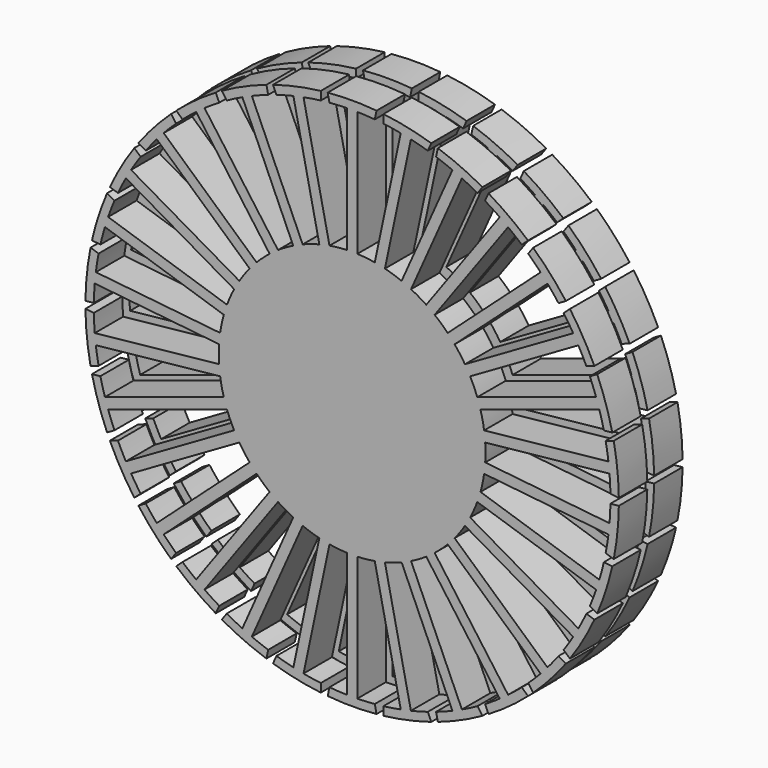
from build123d import *

# Parameters (mm, degrees)
F1_DEPTH = 25.4
F2_R     = 86.282686122
F3_DEPTH = 6.35
F5_DEPTH = 25.4


# Not quite as in the source:
# - a feature names something its author has since deleted; it is built from what else it names


with BuildPart() as f1:
    # F0 (on Front) → F1 (new body)
    with BuildSketch(Plane.XZ):
        with BuildLine():
            Line((16.1989831222, 183.765304664), (17.4450667429, 189.6995509914))
            ThreePointArc((17.4450667429, 189.6995509914), (0, 190.5), (-17.4450667429, 189.6995509914))
            Line((-17.4450667429, 189.6995509914), (-16.1989831222, 183.765304664))
            ThreePointArc((-16.1989831222, 183.765304664), (-9.9568666377, 184.2089983122), (-3.7032927424, 184.4407218466))
            Line((-3.7032927424, 184.4407218466), (-3.7032927424, 95.1779812922))
            ThreePointArc((-3.7032927424, 95.1779812922), (-9.9563361262, 94.7282105338), (-16.1662481083, 93.8680718993))
            ThreePointArc((-16.1662481083, 93.8680718993), (-19.8035885504, 93.1685589699), (-23.4109819298, 92.328156188))
            ThreePointArc((-23.4109819298, 92.328156188), (-29.4338687142, 90.5881331771), (-35.3292463424, 88.4556773355))
            ThreePointArc((-35.3292463424, 88.4556773355), (-38.741665253, 87.0152048405), (-42.0954988686, 85.4431476188))
            ThreePointArc((-42.0954988686, 85.4431476188), (-47.625, 82.4889197105), (-52.9481869828, 79.1773452146))
            ThreePointArc((-52.9481869828, 79.1773452146), (-55.9865452809, 77.0588687142), (-58.9402405103, 74.8238634968))
            ThreePointArc((-58.9402405103, 74.8238634968), (-63.7346902557, 70.7845446267), (-68.2530377785, 66.4385831728))
            ThreePointArc((-68.2530377785, 66.4385831728), (-70.7845446267, 63.7346902557), (-73.2090108149, 60.9344174954))
            ThreePointArc((-73.2090108149, 60.9344174954), (-77.0588687142, 55.9865452809), (-80.5749033088, 50.7961362387))
            ThreePointArc((-80.5749033088, 50.7961362387), (-82.4889197105, 47.625), (-84.2781960512, 44.3818450536))
            ThreePointArc((-84.2781960512, 44.3818450536), (-87.0152048405, 38.741665253), (-89.3752589233, 32.933654404))
            ThreePointArc((-89.3752589233, 32.933654404), (-90.5881331771, 29.4338687142), (-91.6640197083, 25.8895730152))
            ThreePointArc((-91.6640197083, 25.8895730152), (-93.1685589699, 19.8035885504), (-94.2694868527, 13.6318138386))
            ThreePointArc((-94.2694868527, 13.6318138386), (-94.7282105338, 9.9563361262), (-95.0436858515, 6.2658024042))
            ThreePointArc((-95.0436858515, 6.2658024042), (-95.25, 0), (-95.0436858515, -6.2658024042))
            ThreePointArc((-95.0436858515, -6.2658024042), (-94.7282105338, -9.9563361262), (-94.2694868527, -13.6318138386))
            ThreePointArc((-94.2694868527, -13.6318138386), (-93.1685589699, -19.8035885504), (-91.6640197083, -25.8895730152))
            ThreePointArc((-91.6640197083, -25.8895730152), (-90.5881331771, -29.4338687142), (-89.3752589233, -32.933654404))
            ThreePointArc((-89.3752589233, -32.933654404), (-87.0152048405, -38.741665253), (-84.2781960512, -44.3818450536))
            ThreePointArc((-84.2781960512, -44.3818450536), (-82.4889197105, -47.625), (-80.5749033088, -50.7961362387))
            ThreePointArc((-80.5749033088, -50.7961362387), (-77.0588687142, -55.9865452809), (-73.2090108149, -60.9344174954))
            ThreePointArc((-73.2090108149, -60.9344174954), (-70.7845446267, -63.7346902557), (-68.2530377785, -66.4385831728))
            ThreePointArc((-68.2530377785, -66.4385831728), (-63.7346902557, -70.7845446267), (-58.9402405103, -74.8238634968))
            ThreePointArc((-58.9402405103, -74.8238634968), (-55.9865452809, -77.0588687142), (-52.9481869828, -79.1773452146))
            ThreePointArc((-52.9481869828, -79.1773452146), (-47.625, -82.4889197105), (-42.0954988686, -85.4431476188))
            ThreePointArc((-42.0954988686, -85.4431476188), (-38.741665253, -87.0152048405), (-35.3292463424, -88.4556773355))
            ThreePointArc((-35.3292463424, -88.4556773355), (-29.4338687142, -90.5881331771), (-23.4109819298, -92.328156188))
            ThreePointArc((-23.4109819298, -92.328156188), (-19.8035885504, -93.1685589699), (-16.1662481083, -93.8680718993))
            ThreePointArc((-16.1662481083, -93.8680718993), (-9.9563361262, -94.7282105338), (-3.7032927424, -95.1779812922))
            ThreePointArc((-3.7032927424, -95.1779812922), (0, -95.25), (3.7032927424, -95.1779812922))
            ThreePointArc((3.7032927424, -95.1779812922), (9.9563361262, -94.7282105338), (16.1662481083, -93.8680718993))
            ThreePointArc((16.1662481083, -93.8680718993), (19.8035885504, -93.1685589699), (23.4109819298, -92.328156188))
            ThreePointArc((23.4109819298, -92.328156188), (29.4338687142, -90.5881331771), (35.3292463424, -88.4556773355))
            ThreePointArc((35.3292463424, -88.4556773355), (38.741665253, -87.0152048405), (42.0954988686, -85.4431476188))
            ThreePointArc((42.0954988686, -85.4431476188), (47.625, -82.4889197105), (52.9481869828, -79.1773452146))
            ThreePointArc((52.9481869828, -79.1773452146), (55.9865452809, -77.0588687142), (58.9402405103, -74.8238634968))
            ThreePointArc((58.9402405103, -74.8238634968), (63.7346902557, -70.7845446267), (68.2530377785, -66.4385831728))
            ThreePointArc((68.2530377785, -66.4385831728), (70.7845446267, -63.7346902557), (73.2090108149, -60.9344174954))
            ThreePointArc((73.2090108149, -60.9344174954), (77.0588687142, -55.9865452809), (80.5749033088, -50.7961362387))
            ThreePointArc((80.5749033088, -50.7961362387), (82.4889197105, -47.625), (84.2781960512, -44.3818450536))
            ThreePointArc((84.2781960512, -44.3818450536), (87.0152048405, -38.741665253), (89.3752589233, -32.933654404))
            ThreePointArc((89.3752589233, -32.933654404), (90.5881331771, -29.4338687142), (91.6640197083, -25.8895730152))
            ThreePointArc((91.6640197083, -25.8895730152), (93.1685589699, -19.8035885504), (94.2694868527, -13.6318138386))
            ThreePointArc((94.2694868527, -13.6318138386), (94.7282105338, -9.9563361262), (95.0436858515, -6.2658024042))
            ThreePointArc((95.0436858515, -6.2658024042), (95.25, 0), (95.0436858515, 6.2658024042))
            ThreePointArc((95.0436858515, 6.2658024042), (94.7282105338, 9.9563361262), (94.2694868527, 13.6318138386))
            ThreePointArc((94.2694868527, 13.6318138386), (93.1685589699, 19.8035885504), (91.6640197083, 25.8895730152))
            ThreePointArc((91.6640197083, 25.8895730152), (90.5881331771, 29.4338687142), (89.3752589233, 32.933654404))
            ThreePointArc((89.3752589233, 32.933654404), (87.0152048405, 38.741665253), (84.2781960512, 44.3818450536))
            ThreePointArc((84.2781960512, 44.3818450536), (82.4889197105, 47.625), (80.5749033088, 50.7961362387))
            ThreePointArc((80.5749033088, 50.7961362387), (77.0588687142, 55.9865452809), (73.2090108149, 60.9344174954))
            ThreePointArc((73.2090108149, 60.9344174954), (70.7845446267, 63.7346902557), (68.2530377785, 66.4385831728))
            ThreePointArc((68.2530377785, 66.4385831728), (63.7346902557, 70.7845446267), (58.9402405103, 74.8238634968))
            ThreePointArc((58.9402405103, 74.8238634968), (55.9865452809, 77.0588687142), (52.9481869828, 79.1773452146))
            ThreePointArc((52.9481869828, 79.1773452146), (47.625, 82.4889197105), (42.0954988686, 85.4431476188))
            ThreePointArc((42.0954988686, 85.4431476188), (38.741665253, 87.0152048405), (35.3292463424, 88.4556773355))
            ThreePointArc((35.3292463424, 88.4556773355), (29.4338687142, 90.5881331771), (23.4109819298, 92.328156188))
            ThreePointArc((23.4109819298, 92.328156188), (19.8035885504, 93.1685589699), (16.1662481083, 93.8680718993))
            ThreePointArc((16.1662481083, 93.8680718993), (9.9563361262, 94.7282105338), (3.7032927424, 95.1779812922))
            Line((3.7032927424, 95.1779812922), (3.7032927424, 184.4407218466))
            ThreePointArc((3.7032927424, 184.4407218466), (9.9568666377, 184.2089983122), (16.1989831222, 183.765304664))
        make_face()
        with BuildLine():
            ThreePointArc((-23.4109819298, 92.328156188), (-19.8035885504, 93.1685589699), (-16.1662481083, 93.8680718993))
            Line((-16.1662481083, 93.8680718993), (-34.725015424, 181.1802074075))
            ThreePointArc((-34.725015424, 181.1802074075), (-28.5599190905, 182.2537387106), (-22.361958731, 183.1175498257))
            Line((-22.361958731, 183.1175498257), (-22.3769042148, 189.1811939855))
            ThreePointArc((-22.3769042148, 189.1811939855), (-39.6071771008, 186.3371179398), (-56.5046045732, 181.9271273396))
            Line((-56.5046045732, 181.9271273396), (-54.0519516817, 176.3816338847))
            ThreePointArc((-54.0519516817, 176.3816338847), (-48.0384895154, 178.1134407548), (-41.9697492455, 179.6402916962))
            Line((-41.9697492455, 179.6402916962), (-23.4109819298, 92.328156188))
        make_face()
        with BuildLine():
            Line((34.725015424, 181.1802074075), (16.1662481083, 93.8680718993))
            ThreePointArc((16.1662481083, 93.8680718993), (19.8035885504, 93.1685589699), (23.4109819298, 92.328156188))
            Line((23.4109819298, 92.328156188), (41.9697492455, 179.6402916962))
            ThreePointArc((41.9697492455, 179.6402916962), (48.0384895154, 178.1134407548), (54.0519516817, 176.3816338847))
            Line((54.0519516817, 176.3816338847), (56.5046045732, 181.9271273396))
            ThreePointArc((56.5046045732, 181.9271273396), (39.6071771008, 186.3371179398), (22.3769042148, 189.1811939855))
            Line((22.3769042148, 189.1811939855), (22.361958731, 183.1175498257))
            ThreePointArc((22.361958731, 183.1175498257), (28.5599190905, 182.2537387106), (34.725015424, 181.1802074075))
        make_face()
        with BuildLine():
            Line((71.6356737873, 170.0012485057), (35.3292463424, 88.4556773355))
            ThreePointArc((35.3292463424, 88.4556773355), (38.741665253, 87.0152048405), (42.0954988686, 85.4431476188))
            Line((42.0954988686, 85.4431476188), (78.4019263135, 166.9887187889))
            ThreePointArc((78.4019263135, 166.9887187889), (84.0205998871, 164.2334711533), (89.5425905826, 161.2892393317))
            Line((89.5425905826, 161.2892393317), (93.0946200445, 166.2036152398))
            ThreePointArc((93.0946200445, 166.2036152398), (77.4833305059, 174.0304096809), (61.2208970819, 180.3947110103))
            Line((61.2208970819, 180.3947110103), (59.9455756831, 174.4666793645))
            ThreePointArc((59.9455756831, 174.4666793645), (65.8284993087, 172.3331161768), (71.6356737873, 170.0012485057))
        make_face()
        with BuildLine():
            Line((105.4155094599, 151.3924192876), (52.9481869828, 79.1773452146))
            ThreePointArc((52.9481869828, 79.1773452146), (55.9865452809, 77.0588687142), (58.9402405103, 74.8238634968))
            Line((58.9402405103, 74.8238634968), (111.4075629873, 147.0389375698))
            ThreePointArc((111.4075629873, 147.0389375698), (116.3306068681, 143.1757107827), (121.119788602, 139.1477310683))
            Line((121.119788602, 139.1477310683), (125.6159539023, 143.2162076206))
            ThreePointArc((125.6159539023, 143.2162076206), (111.9730905617, 154.1177374284), (97.3892429762, 163.7241135341))
            Line((97.3892429762, 163.7241135341), (94.909283327, 158.190777831))
            ThreePointArc((94.909283327, 158.190777831), (100.2200582269, 154.88070952), (105.4155094599, 151.3924192876))
        make_face()
        with BuildLine():
            Line((134.5881815294, 126.1670148852), (68.2530377785, 66.4385831728))
            ThreePointArc((68.2530377785, 66.4385831728), (70.7845446267, 63.7346902557), (73.2090108149, 60.9344174954))
            Line((73.2090108149, 60.9344174954), (139.5441545659, 120.6628492078))
            ThreePointArc((139.5441545659, 120.6628492078), (143.5564081128, 115.8604848177), (147.4034706623, 110.9247992522))
            Line((147.4034706623, 110.9247992522), (152.6472678023, 113.9695645008))
            ThreePointArc((152.6472678023, 113.9695645008), (141.5690892534, 127.4693805114), (129.301211627, 139.897986661))
            Line((129.301211627, 139.897986661), (125.7249998643, 135.0011802228))
            ThreePointArc((125.7249998643, 135.0011802228), (130.2315196914, 130.6592726572), (134.5881815294, 126.1670148852))
        make_face()
        with BuildLine():
            Line((157.8787042403, 95.4275065158), (80.5749033088, 50.7961362387))
            ThreePointArc((80.5749033088, 50.7961362387), (82.4889197105, 47.625), (84.2781960512, 44.3818450536))
            Line((84.2781960512, 44.3818450536), (161.5819969827, 89.0132153308))
            ThreePointArc((161.5819969827, 89.0132153308), (164.5081054629, 83.4815997058), (167.2449137343, 77.8539214327))
            Line((167.2449137343, 77.8539214327), (173.0071636165, 79.7419045256))
            ThreePointArc((173.0071636165, 79.7419045256), (164.9778394209, 95.25), (155.5620968736, 109.9576464658))
            Line((155.5620968736, 109.9576464658), (151.0459306121, 105.9113832313))
            ThreePointArc((151.0459306121, 105.9113832313), (154.5512388252, 100.7273986064), (157.8787042403, 95.4275065158))
        make_face()
        with BuildLine():
            Line((174.2691699899, 60.5173581998), (89.3752589233, 32.933654404))
            ThreePointArc((89.3752589233, 32.933654404), (90.5881331771, 29.4338687142), (91.6640197083, 25.8895730152))
            Line((91.6640197083, 25.8895730152), (176.5579307749, 53.473276811))
            ThreePointArc((176.5579307749, 53.473276811), (178.2700092068, 47.4541680976), (179.776951546, 41.3804536619))
            Line((179.776951546, 41.3804536619), (185.8058162002, 42.0291406786))
            ThreePointArc((185.8058162002, 42.0291406786), (181.1762663542, 58.8677374284), (175.0241720171, 75.2116294847))
            Line((175.0241720171, 75.2116294847), (169.7654293933, 72.1927505734))
            ThreePointArc((169.7654293933, 72.1927505734), (172.1163272033, 66.3932538929), (174.2691699899, 60.5173581998))
        make_face()
        with BuildLine():
            Line((183.0432367746, 22.9623109358), (94.2694868527, 13.6318138386))
            ThreePointArc((94.2694868527, 13.6318138386), (94.7282105338, 9.9563361262), (95.0436858515, 6.2658024042))
            Line((95.0436858515, 6.2658024042), (183.8174357734, 15.5962995014))
            ThreePointArc((183.8174357734, 15.5962995014), (184.240658114, 9.3527616332), (184.4518739096, 3.0984615007))
            Line((184.4518739096, 3.0984615007), (190.4838630207, 2.4795017057))
            ThreePointArc((190.4838630207, 2.4795017057), (189.4564210677, 19.9126722525), (186.8368509842, 37.1785033897))
            Line((186.8368509842, 37.1785033897), (181.0653642851, 35.3189482962))
            ThreePointArc((181.0653642851, 35.3189482962), (182.1591061768, 29.1574053941), (183.0432367746, 22.9623109358))
        make_face()
        with BuildLine():
            Line((183.8174357734, -15.5962995014), (95.0436858515, -6.2658024042))
            ThreePointArc((95.0436858515, -6.2658024042), (94.7282105338, -9.9563361262), (94.2694868527, -13.6318138386))
            Line((94.2694868527, -13.6318138386), (183.0432367746, -22.9623109358))
            ThreePointArc((183.0432367746, -22.9623109358), (182.1591061768, -29.1574053941), (181.0653642851, -35.3189482962))
            Line((181.0653642851, -35.3189482962), (186.8368509842, -37.1785033897))
            ThreePointArc((186.8368509842, -37.1785033897), (189.4564210677, -19.9126722525), (190.4838630207, -2.4795017057))
            Line((190.4838630207, -2.4795017057), (184.4518739096, -3.0984615007))
            ThreePointArc((184.4518739096, -3.0984615007), (184.240658114, -9.3527616332), (183.8174357734, -15.5962995014))
        make_face()
        with BuildLine():
            Line((176.5579307749, -53.473276811), (91.6640197083, -25.8895730152))
            ThreePointArc((91.6640197083, -25.8895730152), (90.5881331771, -29.4338687142), (89.3752589233, -32.933654404))
            Line((89.3752589233, -32.933654404), (174.2691699899, -60.5173581998))
            ThreePointArc((174.2691699899, -60.5173581998), (172.1163272033, -66.3932538929), (169.7654293933, -72.1927505734))
            Line((169.7654293933, -72.1927505734), (175.0241720171, -75.2116294847))
            ThreePointArc((175.0241720171, -75.2116294847), (181.1762663542, -58.8677374284), (185.8058162002, -42.0291406786))
            Line((185.8058162002, -42.0291406786), (179.776951546, -41.3804536619))
            ThreePointArc((179.776951546, -41.3804536619), (178.2700092068, -47.4541680976), (176.5579307749, -53.473276811))
        make_face()
        with BuildLine():
            Line((161.5819969827, -89.0132153308), (84.2781960512, -44.3818450536))
            ThreePointArc((84.2781960512, -44.3818450536), (82.4889197105, -47.625), (80.5749033088, -50.7961362387))
            Line((80.5749033088, -50.7961362387), (157.8787042403, -95.4275065158))
            ThreePointArc((157.8787042403, -95.4275065158), (154.5512388252, -100.7273986064), (151.0459306121, -105.9113832313))
            Line((151.0459306121, -105.9113832313), (155.5620968736, -109.9576464658))
            ThreePointArc((155.5620968736, -109.9576464658), (164.9778394209, -95.25), (173.0071636165, -79.7419045256))
            Line((173.0071636165, -79.7419045256), (167.2449137343, -77.8539214327))
            ThreePointArc((167.2449137343, -77.8539214327), (164.5081054629, -83.4815997058), (161.5819969827, -89.0132153308))
        make_face()
        with BuildLine():
            Line((139.5441545659, -120.6628492078), (73.2090108149, -60.9344174954))
            ThreePointArc((73.2090108149, -60.9344174954), (70.7845446267, -63.7346902557), (68.2530377785, -66.4385831728))
            Line((68.2530377785, -66.4385831728), (134.5881815294, -126.1670148852))
            ThreePointArc((134.5881815294, -126.1670148852), (130.2315196914, -130.6592726572), (125.7249998643, -135.0011802228))
            Line((125.7249998643, -135.0011802228), (129.301211627, -139.897986661))
            ThreePointArc((129.301211627, -139.897986661), (141.5690892534, -127.4693805114), (152.6472678023, -113.9695645008))
            Line((152.6472678023, -113.9695645008), (147.4034706623, -110.9247992522))
            ThreePointArc((147.4034706623, -110.9247992522), (143.5564081128, -115.8604848177), (139.5441545659, -120.6628492078))
        make_face()
        with BuildLine():
            Line((111.4075629873, -147.0389375698), (58.9402405103, -74.8238634968))
            ThreePointArc((58.9402405103, -74.8238634968), (55.9865452809, -77.0588687142), (52.9481869828, -79.1773452146))
            Line((52.9481869828, -79.1773452146), (105.4155094599, -151.3924192876))
            ThreePointArc((105.4155094599, -151.3924192876), (100.2200582269, -154.88070952), (94.909283327, -158.190777831))
            Line((94.909283327, -158.190777831), (97.3892429762, -163.7241135341))
            ThreePointArc((97.3892429762, -163.7241135341), (111.9730905617, -154.1177374284), (125.6159539023, -143.2162076206))
            Line((125.6159539023, -143.2162076206), (121.119788602, -139.1477310683))
            ThreePointArc((121.119788602, -139.1477310683), (116.3306068681, -143.1757107827), (111.4075629873, -147.0389375698))
        make_face()
        with BuildLine():
            Line((78.4019263135, -166.9887187889), (42.0954988686, -85.4431476188))
            ThreePointArc((42.0954988686, -85.4431476188), (38.741665253, -87.0152048405), (35.3292463424, -88.4556773355))
            Line((35.3292463424, -88.4556773355), (71.6356737873, -170.0012485057))
            ThreePointArc((71.6356737873, -170.0012485057), (65.8284993087, -172.3331161768), (59.9455756831, -174.4666793645))
            Line((59.9455756831, -174.4666793645), (61.2208970819, -180.3947110103))
            ThreePointArc((61.2208970819, -180.3947110103), (77.4833305059, -174.0304096809), (93.0946200445, -166.2036152398))
            Line((93.0946200445, -166.2036152398), (89.5425905826, -161.2892393317))
            ThreePointArc((89.5425905826, -161.2892393317), (84.0205998871, -164.2334711533), (78.4019263135, -166.9887187889))
        make_face()
        with BuildLine():
            Line((41.9697492455, -179.6402916962), (23.4109819298, -92.328156188))
            ThreePointArc((23.4109819298, -92.328156188), (19.8035885504, -93.1685589699), (16.1662481083, -93.8680718993))
            Line((16.1662481083, -93.8680718993), (34.725015424, -181.1802074075))
            ThreePointArc((34.725015424, -181.1802074075), (28.5599190905, -182.2537387106), (22.361958731, -183.1175498257))
            Line((22.361958731, -183.1175498257), (22.3769042148, -189.1811939855))
            ThreePointArc((22.3769042148, -189.1811939855), (39.6071771008, -186.3371179398), (56.5046045732, -181.9271273396))
            Line((56.5046045732, -181.9271273396), (54.0519516817, -176.3816338847))
            ThreePointArc((54.0519516817, -176.3816338847), (48.0384895154, -178.1134407548), (41.9697492455, -179.6402916962))
        make_face()
        with BuildLine():
            Line((3.7032927424, -184.4407218466), (3.7032927424, -95.1779812922))
            ThreePointArc((3.7032927424, -95.1779812922), (0, -95.25), (-3.7032927424, -95.1779812922))
            Line((-3.7032927424, -95.1779812922), (-3.7032927424, -184.4407218466))
            ThreePointArc((-3.7032927424, -184.4407218466), (-9.9568666377, -184.2089983122), (-16.1989831222, -183.765304664))
            Line((-16.1989831222, -183.765304664), (-17.4450667429, -189.6995509914))
            ThreePointArc((-17.4450667429, -189.6995509914), (0, -190.5), (17.4450667429, -189.6995509914))
            Line((17.4450667429, -189.6995509914), (16.1989831222, -183.765304664))
            ThreePointArc((16.1989831222, -183.765304664), (9.9568666377, -184.2089983122), (3.7032927424, -184.4407218466))
        make_face()
        with BuildLine():
            ThreePointArc((-16.1662481083, -93.8680718993), (-19.8035885504, -93.1685589699), (-23.4109819298, -92.328156188))
            Line((-23.4109819298, -92.328156188), (-41.9697492455, -179.6402916962))
            ThreePointArc((-41.9697492455, -179.6402916962), (-48.0384895154, -178.1134407548), (-54.0519516817, -176.3816338847))
            Line((-54.0519516817, -176.3816338847), (-56.5046045732, -181.9271273396))
            ThreePointArc((-56.5046045732, -181.9271273396), (-39.6071771008, -186.3371179398), (-22.3769042148, -189.1811939855))
            Line((-22.3769042148, -189.1811939855), (-22.361958731, -183.1175498257))
            ThreePointArc((-22.361958731, -183.1175498257), (-28.5599190905, -182.2537387106), (-34.725015424, -181.1802074075))
            Line((-34.725015424, -181.1802074075), (-16.1662481083, -93.8680718993))
        make_face()
        with BuildLine():
            ThreePointArc((-35.3292463424, -88.4556773355), (-38.741665253, -87.0152048405), (-42.0954988686, -85.4431476188))
            Line((-42.0954988686, -85.4431476188), (-78.4019263135, -166.9887187889))
            ThreePointArc((-78.4019263135, -166.9887187889), (-84.0205998871, -164.2334711533), (-89.5425905826, -161.2892393317))
            Line((-89.5425905826, -161.2892393317), (-93.0946200445, -166.2036152398))
            ThreePointArc((-93.0946200445, -166.2036152398), (-77.4833305059, -174.0304096809), (-61.2208970819, -180.3947110103))
            Line((-61.2208970819, -180.3947110103), (-59.9455756831, -174.4666793645))
            ThreePointArc((-59.9455756831, -174.4666793645), (-65.8284993087, -172.3331161768), (-71.6356737873, -170.0012485057))
            Line((-71.6356737873, -170.0012485057), (-35.3292463424, -88.4556773355))
        make_face()
        with BuildLine():
            ThreePointArc((-52.9481869828, -79.1773452146), (-55.9865452809, -77.0588687142), (-58.9402405103, -74.8238634968))
            Line((-58.9402405103, -74.8238634968), (-111.4075629873, -147.0389375698))
            ThreePointArc((-111.4075629873, -147.0389375698), (-116.3306068681, -143.1757107827), (-121.119788602, -139.1477310683))
            Line((-121.119788602, -139.1477310683), (-125.6159539023, -143.2162076206))
            ThreePointArc((-125.6159539023, -143.2162076206), (-111.9730905617, -154.1177374284), (-97.3892429762, -163.7241135341))
            Line((-97.3892429762, -163.7241135341), (-94.909283327, -158.190777831))
            ThreePointArc((-94.909283327, -158.190777831), (-100.2200582269, -154.88070952), (-105.4155094599, -151.3924192876))
            Line((-105.4155094599, -151.3924192876), (-52.9481869828, -79.1773452146))
        make_face()
        with BuildLine():
            ThreePointArc((-68.2530377785, -66.4385831728), (-70.7845446267, -63.7346902557), (-73.2090108149, -60.9344174954))
            Line((-73.2090108149, -60.9344174954), (-139.5441545659, -120.6628492078))
            ThreePointArc((-139.5441545659, -120.6628492078), (-143.5564081128, -115.8604848177), (-147.4034706623, -110.9247992522))
            Line((-147.4034706623, -110.9247992522), (-152.6472678023, -113.9695645008))
            ThreePointArc((-152.6472678023, -113.9695645008), (-141.5690892534, -127.4693805114), (-129.301211627, -139.897986661))
            Line((-129.301211627, -139.897986661), (-125.7249998643, -135.0011802228))
            ThreePointArc((-125.7249998643, -135.0011802228), (-130.2315196914, -130.6592726572), (-134.5881815294, -126.1670148852))
            Line((-134.5881815294, -126.1670148852), (-68.2530377785, -66.4385831728))
        make_face()
        with BuildLine():
            ThreePointArc((-80.5749033088, -50.7961362387), (-82.4889197105, -47.625), (-84.2781960512, -44.3818450536))
            Line((-84.2781960512, -44.3818450536), (-161.5819969827, -89.0132153308))
            ThreePointArc((-161.5819969827, -89.0132153308), (-164.5081054629, -83.4815997058), (-167.2449137343, -77.8539214327))
            Line((-167.2449137343, -77.8539214327), (-173.0071636165, -79.7419045256))
            ThreePointArc((-173.0071636165, -79.7419045256), (-164.9778394209, -95.25), (-155.5620968736, -109.9576464658))
            Line((-155.5620968736, -109.9576464658), (-151.0459306121, -105.9113832313))
            ThreePointArc((-151.0459306121, -105.9113832313), (-154.5512388252, -100.7273986064), (-157.8787042403, -95.4275065158))
            Line((-157.8787042403, -95.4275065158), (-80.5749033088, -50.7961362387))
        make_face()
        with BuildLine():
            ThreePointArc((-89.3752589233, -32.933654404), (-90.5881331771, -29.4338687142), (-91.6640197083, -25.8895730152))
            Line((-91.6640197083, -25.8895730152), (-176.5579307749, -53.473276811))
            ThreePointArc((-176.5579307749, -53.473276811), (-178.2700092068, -47.4541680976), (-179.776951546, -41.3804536619))
            Line((-179.776951546, -41.3804536619), (-185.8058162002, -42.0291406786))
            ThreePointArc((-185.8058162002, -42.0291406786), (-181.1762663542, -58.8677374284), (-175.0241720171, -75.2116294847))
            Line((-175.0241720171, -75.2116294847), (-169.7654293933, -72.1927505734))
            ThreePointArc((-169.7654293933, -72.1927505734), (-172.1163272033, -66.3932538929), (-174.2691699899, -60.5173581998))
            Line((-174.2691699899, -60.5173581998), (-89.3752589233, -32.933654404))
        make_face()
        with BuildLine():
            ThreePointArc((-94.2694868527, -13.6318138386), (-94.7282105338, -9.9563361262), (-95.0436858515, -6.2658024042))
            Line((-95.0436858515, -6.2658024042), (-183.8174357734, -15.5962995014))
            ThreePointArc((-183.8174357734, -15.5962995014), (-184.240658114, -9.3527616332), (-184.4518739096, -3.0984615007))
            Line((-184.4518739096, -3.0984615007), (-190.4838630207, -2.4795017057))
            ThreePointArc((-190.4838630207, -2.4795017057), (-189.4564210677, -19.9126722525), (-186.8368509842, -37.1785033897))
            Line((-186.8368509842, -37.1785033897), (-181.0653642851, -35.3189482962))
            ThreePointArc((-181.0653642851, -35.3189482962), (-182.1591061768, -29.1574053941), (-183.0432367746, -22.9623109358))
            Line((-183.0432367746, -22.9623109358), (-94.2694868527, -13.6318138386))
        make_face()
        with BuildLine():
            ThreePointArc((-95.0436858515, 6.2658024042), (-94.7282105338, 9.9563361262), (-94.2694868527, 13.6318138386))
            Line((-94.2694868527, 13.6318138386), (-183.0432367746, 22.9623109358))
            ThreePointArc((-183.0432367746, 22.9623109358), (-182.1591061768, 29.1574053941), (-181.0653642851, 35.3189482962))
            Line((-181.0653642851, 35.3189482962), (-186.8368509842, 37.1785033897))
            ThreePointArc((-186.8368509842, 37.1785033897), (-189.4564210677, 19.9126722525), (-190.4838630207, 2.4795017057))
            Line((-190.4838630207, 2.4795017057), (-184.4518739096, 3.0984615007))
            ThreePointArc((-184.4518739096, 3.0984615007), (-184.240658114, 9.3527616332), (-183.8174357734, 15.5962995014))
            Line((-183.8174357734, 15.5962995014), (-95.0436858515, 6.2658024042))
        make_face()
        with BuildLine():
            ThreePointArc((-91.6640197083, 25.8895730152), (-90.5881331771, 29.4338687142), (-89.3752589233, 32.933654404))
            Line((-89.3752589233, 32.933654404), (-174.2691699899, 60.5173581998))
            ThreePointArc((-174.2691699899, 60.5173581998), (-172.1163272033, 66.3932538929), (-169.7654293933, 72.1927505734))
            Line((-169.7654293933, 72.1927505734), (-175.0241720171, 75.2116294847))
            ThreePointArc((-175.0241720171, 75.2116294847), (-181.1762663542, 58.8677374284), (-185.8058162002, 42.0291406786))
            Line((-185.8058162002, 42.0291406786), (-179.776951546, 41.3804536619))
            ThreePointArc((-179.776951546, 41.3804536619), (-178.2700092068, 47.4541680976), (-176.5579307749, 53.473276811))
            Line((-176.5579307749, 53.473276811), (-91.6640197083, 25.8895730152))
        make_face()
        with BuildLine():
            ThreePointArc((-84.2781960512, 44.3818450536), (-82.4889197105, 47.625), (-80.5749033088, 50.7961362387))
            Line((-80.5749033088, 50.7961362387), (-157.8787042403, 95.4275065158))
            ThreePointArc((-157.8787042403, 95.4275065158), (-154.5512388252, 100.7273986064), (-151.0459306121, 105.9113832313))
            Line((-151.0459306121, 105.9113832313), (-155.5620968736, 109.9576464658))
            ThreePointArc((-155.5620968736, 109.9576464658), (-164.9778394209, 95.25), (-173.0071636165, 79.7419045256))
            Line((-173.0071636165, 79.7419045256), (-167.2449137343, 77.8539214327))
            ThreePointArc((-167.2449137343, 77.8539214327), (-164.5081054629, 83.4815997058), (-161.5819969827, 89.0132153308))
            Line((-161.5819969827, 89.0132153308), (-84.2781960512, 44.3818450536))
        make_face()
        with BuildLine():
            ThreePointArc((-73.2090108149, 60.9344174954), (-70.7845446267, 63.7346902557), (-68.2530377785, 66.4385831728))
            Line((-68.2530377785, 66.4385831728), (-134.5881815294, 126.1670148852))
            ThreePointArc((-134.5881815294, 126.1670148852), (-130.2315196914, 130.6592726572), (-125.7249998643, 135.0011802228))
            Line((-125.7249998643, 135.0011802228), (-129.301211627, 139.897986661))
            ThreePointArc((-129.301211627, 139.897986661), (-141.5690892534, 127.4693805114), (-152.6472678023, 113.9695645008))
            Line((-152.6472678023, 113.9695645008), (-147.4034706623, 110.9247992522))
            ThreePointArc((-147.4034706623, 110.9247992522), (-143.5564081128, 115.8604848177), (-139.5441545659, 120.6628492078))
            Line((-139.5441545659, 120.6628492078), (-73.2090108149, 60.9344174954))
        make_face()
        with BuildLine():
            ThreePointArc((-58.9402405103, 74.8238634968), (-55.9865452809, 77.0588687142), (-52.9481869828, 79.1773452146))
            Line((-52.9481869828, 79.1773452146), (-105.4155094599, 151.3924192876))
            ThreePointArc((-105.4155094599, 151.3924192876), (-100.2200582269, 154.88070952), (-94.909283327, 158.190777831))
            Line((-94.909283327, 158.190777831), (-97.3892429762, 163.7241135341))
            ThreePointArc((-97.3892429762, 163.7241135341), (-111.9730905617, 154.1177374284), (-125.6159539023, 143.2162076206))
            Line((-125.6159539023, 143.2162076206), (-121.119788602, 139.1477310683))
            ThreePointArc((-121.119788602, 139.1477310683), (-116.3306068681, 143.1757107827), (-111.4075629873, 147.0389375698))
            Line((-111.4075629873, 147.0389375698), (-58.9402405103, 74.8238634968))
        make_face()
        with BuildLine():
            ThreePointArc((-42.0954988686, 85.4431476188), (-38.741665253, 87.0152048405), (-35.3292463424, 88.4556773355))
            Line((-35.3292463424, 88.4556773355), (-71.6356737873, 170.0012485057))
            ThreePointArc((-71.6356737873, 170.0012485057), (-65.8284993087, 172.3331161768), (-59.9455756831, 174.4666793645))
            Line((-59.9455756831, 174.4666793645), (-61.2208970819, 180.3947110103))
            ThreePointArc((-61.2208970819, 180.3947110103), (-77.4833305059, 174.0304096809), (-93.0946200445, 166.2036152398))
            Line((-93.0946200445, 166.2036152398), (-89.5425905826, 161.2892393317))
            ThreePointArc((-89.5425905826, 161.2892393317), (-84.0205998871, 164.2334711533), (-78.4019263135, 166.9887187889))
            Line((-78.4019263135, 166.9887187889), (-42.0954988686, 85.4431476188))
        make_face()
    extrude(amount=F1_DEPTH)

    # F2 (on face) → F3 (join)
    with BuildSketch(Plane.XZ.offset(25.4)):
        Circle(F2_R)
    extrude(amount=F3_DEPTH)

    # F4 (on face) → F5 (join)
    with BuildSketch(Plane.XZ.offset(31.75)):
        with BuildLine():
            Line((16.3894969565, 182.7363048395), (17.6355805772, 188.6705511669))
            ThreePointArc((17.6355805772, 188.6705511669), (0.1905138342, 189.4710001755), (-17.2545529087, 188.6705511669))
            Line((-17.2545529087, 188.6705511669), (-16.008469288, 182.7363048395))
            ThreePointArc((-16.008469288, 182.7363048395), (-9.7663528034, 183.1799984878), (-3.5127789081, 183.4117220222))
            Line((-3.5127789081, 183.4117220222), (-3.5127789081, 94.1489814678))
            ThreePointArc((-3.5127789081, 94.1489814678), (-9.765822292, 93.6992107094), (-15.9757342741, 92.8390720749))
            ThreePointArc((-15.9757342741, 92.8390720749), (-19.6130747162, 92.1395591454), (-23.2204680956, 91.2991563636))
            ThreePointArc((-23.2204680956, 91.2991563636), (-29.24335488, 89.5591333527), (-35.1387325082, 87.426677511))
            ThreePointArc((-35.1387325082, 87.426677511), (-38.5511514187, 85.986205016), (-41.9049850344, 84.4141477943))
            ThreePointArc((-41.9049850344, 84.4141477943), (-47.4344861658, 81.459919886), (-52.7576731486, 78.1483453901))
            ThreePointArc((-52.7576731486, 78.1483453901), (-55.7960314466, 76.0298688898), (-58.749726676, 73.7948636724))
            ThreePointArc((-58.749726676, 73.7948636724), (-63.5441764214, 69.7555448023), (-68.0625239442, 65.4095833483))
            ThreePointArc((-68.0625239442, 65.4095833483), (-70.5940307925, 62.7056904312), (-73.0184969807, 59.9054176709))
            ThreePointArc((-73.0184969807, 59.9054176709), (-76.86835488, 54.9575454564), (-80.3843894746, 49.7671364142))
            ThreePointArc((-80.3843894746, 49.7671364142), (-82.2984058762, 46.5960001755), (-84.0876822169, 43.3528452291))
            ThreePointArc((-84.0876822169, 43.3528452291), (-86.8246910062, 37.7126654285), (-89.184745089, 31.9046545795))
            ThreePointArc((-89.184745089, 31.9046545795), (-90.3976193429, 28.4048688898), (-91.4735058741, 24.8605731908))
            ThreePointArc((-91.4735058741, 24.8605731908), (-92.9780451357, 18.7745887259), (-94.0789730184, 12.6028140142))
            ThreePointArc((-94.0789730184, 12.6028140142), (-94.5376966996, 8.9273363018), (-94.8531720172, 5.2368025797))
            ThreePointArc((-94.8531720172, 5.2368025797), (-95.0594861658, -1.0289998245), (-94.8531720172, -7.2948022286))
            ThreePointArc((-94.8531720172, -7.2948022286), (-94.5376966996, -10.9853359507), (-94.0789730184, -14.6608136631))
            ThreePointArc((-94.0789730184, -14.6608136631), (-92.9780451357, -20.8325883748), (-91.4735058741, -26.9185728397))
            ThreePointArc((-91.4735058741, -26.9185728397), (-90.3976193429, -30.4628685387), (-89.184745089, -33.9626542284))
            ThreePointArc((-89.184745089, -33.9626542284), (-86.8246910062, -39.7706650774), (-84.0876822169, -45.410844878))
            ThreePointArc((-84.0876822169, -45.410844878), (-82.2984058762, -48.6539998245), (-80.3843894746, -51.8251360631))
            ThreePointArc((-80.3843894746, -51.8251360631), (-76.86835488, -57.0155451053), (-73.0184969807, -61.9634173198))
            ThreePointArc((-73.0184969807, -61.9634173198), (-70.5940307925, -64.7636900801), (-68.0625239442, -67.4675829972))
            ThreePointArc((-68.0625239442, -67.4675829972), (-63.5441764214, -71.8135444512), (-58.749726676, -75.8528633213))
            ThreePointArc((-58.749726676, -75.8528633213), (-55.7960314466, -78.0878685387), (-52.7576731486, -80.2063450391))
            ThreePointArc((-52.7576731486, -80.2063450391), (-47.4344861658, -83.5179195349), (-41.9049850344, -86.4721474432))
            ThreePointArc((-41.9049850344, -86.4721474432), (-38.5511514187, -88.0442046649), (-35.1387325082, -89.4846771599))
            ThreePointArc((-35.1387325082, -89.4846771599), (-29.24335488, -91.6171330016), (-23.2204680956, -93.3571560125))
            ThreePointArc((-23.2204680956, -93.3571560125), (-19.6130747162, -94.1975587943), (-15.9757342741, -94.8970717238))
            ThreePointArc((-15.9757342741, -94.8970717238), (-9.765822292, -95.7572103583), (-3.5127789081, -96.2069811167))
            ThreePointArc((-3.5127789081, -96.2069811167), (0.1905138342, -96.2789998245), (3.8938065766, -96.2069811167))
            ThreePointArc((3.8938065766, -96.2069811167), (10.1468499605, -95.7572103583), (16.3567619426, -94.8970717238))
            ThreePointArc((16.3567619426, -94.8970717238), (19.9941023846, -94.1975587943), (23.6014957641, -93.3571560125))
            ThreePointArc((23.6014957641, -93.3571560125), (29.6243825485, -91.6171330016), (35.5197601767, -89.4846771599))
            ThreePointArc((35.5197601767, -89.4846771599), (38.9321790872, -88.0442046649), (42.2860127029, -86.4721474432))
            ThreePointArc((42.2860127029, -86.4721474432), (47.8155138342, -83.5179195349), (53.1387008171, -80.2063450391))
            ThreePointArc((53.1387008171, -80.2063450391), (56.1770591151, -78.0878685387), (59.1307543445, -75.8528633213))
            ThreePointArc((59.1307543445, -75.8528633213), (63.9252040899, -71.8135444512), (68.4435516127, -67.4675829973))
            ThreePointArc((68.4435516127, -67.4675829973), (70.975058461, -64.7636900801), (73.3995246492, -61.9634173198))
            ThreePointArc((73.3995246492, -61.9634173198), (77.2493825485, -57.0155451053), (80.7654171431, -51.8251360631))
            ThreePointArc((80.7654171431, -51.8251360631), (82.6794335447, -48.6539998245), (84.4687098854, -45.410844878))
            ThreePointArc((84.4687098854, -45.410844878), (87.2057186747, -39.7706650774), (89.5657727575, -33.9626542284))
            ThreePointArc((89.5657727575, -33.9626542284), (90.7786470114, -30.4628685387), (91.8545335426, -26.9185728397))
            ThreePointArc((91.8545335426, -26.9185728397), (93.3590728041, -20.8325883748), (94.4600006869, -14.6608136631))
            ThreePointArc((94.4600006869, -14.6608136631), (94.9187243681, -10.9853359507), (95.2341996857, -7.2948022286))
            ThreePointArc((95.2341996857, -7.2948022286), (95.4405138342, -1.0289998245), (95.2341996857, 5.2368025797))
            ThreePointArc((95.2341996857, 5.2368025797), (94.9187243681, 8.9273363018), (94.4600006869, 12.6028140142))
            ThreePointArc((94.4600006869, 12.6028140142), (93.3590728041, 18.7745887259), (91.8545335426, 24.8605731908))
            ThreePointArc((91.8545335426, 24.8605731908), (90.7786470114, 28.4048688898), (89.5657727575, 31.9046545795))
            ThreePointArc((89.5657727575, 31.9046545795), (87.2057186747, 37.7126654285), (84.4687098854, 43.3528452291))
            ThreePointArc((84.4687098854, 43.3528452291), (82.6794335447, 46.5960001755), (80.7654171431, 49.7671364142))
            ThreePointArc((80.7654171431, 49.7671364142), (77.2493825485, 54.9575454564), (73.3995246492, 59.9054176709))
            ThreePointArc((73.3995246492, 59.9054176709), (70.975058461, 62.7056904312), (68.4435516127, 65.4095833483))
            ThreePointArc((68.4435516127, 65.4095833483), (63.9252040899, 69.7555448023), (59.1307543445, 73.7948636724))
            ThreePointArc((59.1307543445, 73.7948636724), (56.1770591151, 76.0298688898), (53.1387008171, 78.1483453901))
            ThreePointArc((53.1387008171, 78.1483453901), (47.8155138342, 81.459919886), (42.2860127029, 84.4141477943))
            ThreePointArc((42.2860127029, 84.4141477943), (38.9321790872, 85.986205016), (35.5197601767, 87.426677511))
            ThreePointArc((35.5197601767, 87.426677511), (29.6243825485, 89.5591333527), (23.6014957641, 91.2991563636))
            ThreePointArc((23.6014957641, 91.2991563636), (19.9941023846, 92.1395591454), (16.3567619426, 92.8390720749))
            ThreePointArc((16.3567619426, 92.8390720749), (10.1468499605, 93.6992107094), (3.8938065766, 94.1489814678))
            Line((3.8938065766, 94.1489814678), (3.8938065766, 183.4117220222))
            ThreePointArc((3.8938065766, 183.4117220222), (10.1473804719, 183.1799984878), (16.3894969565, 182.7363048395))
        make_face()
        with BuildLine():
            Line((34.9155292583, 180.1512075831), (16.3567619426, 92.8390720749))
            ThreePointArc((16.3567619426, 92.8390720749), (19.9941023846, 92.1395591454), (23.6014957641, 91.2991563636))
            Line((23.6014957641, 91.2991563636), (42.1602630798, 178.6112918718))
            ThreePointArc((42.1602630798, 178.6112918718), (48.2290033496, 177.0844409304), (54.2424655159, 175.3526340603))
            Line((54.2424655159, 175.3526340603), (56.6951184075, 180.8981275151))
            ThreePointArc((56.6951184075, 180.8981275151), (39.797690935, 185.3081181153), (22.567418049, 188.152194161))
            Line((22.567418049, 188.152194161), (22.5524725652, 182.0885500012))
            ThreePointArc((22.5524725652, 182.0885500012), (28.7504329247, 181.2247388861), (34.9155292583, 180.1512075831))
        make_face()
        with BuildLine():
            ThreePointArc((-23.2204680956, 91.2991563636), (-19.6130747162, 92.1395591454), (-15.9757342741, 92.8390720749))
            Line((-15.9757342741, 92.8390720749), (-34.5345015898, 180.1512075831))
            ThreePointArc((-34.5345015898, 180.1512075831), (-28.3694052562, 181.2247388861), (-22.1714448967, 182.0885500012))
            Line((-22.1714448967, 182.0885500012), (-22.1863903805, 188.152194161))
            ThreePointArc((-22.1863903805, 188.152194161), (-39.4166632665, 185.3081181153), (-56.314090739, 180.8981275151))
            Line((-56.314090739, 180.8981275151), (-53.8614378474, 175.3526340603))
            ThreePointArc((-53.8614378474, 175.3526340603), (-47.8479756812, 177.0844409304), (-41.7792354113, 178.6112918718))
            Line((-41.7792354113, 178.6112918718), (-23.2204680956, 91.2991563636))
        make_face()
        with BuildLine():
            Line((71.8261876215, 168.9722486812), (35.5197601767, 87.426677511))
            ThreePointArc((35.5197601767, 87.426677511), (38.9321790872, 85.986205016), (42.2860127029, 84.4141477943))
            Line((42.2860127029, 84.4141477943), (78.5924401477, 165.9597189645))
            ThreePointArc((78.5924401477, 165.9597189645), (84.2111137213, 163.2044713288), (89.7331044168, 160.2602395072))
            Line((89.7331044168, 160.2602395072), (93.2851338787, 165.1746154153))
            ThreePointArc((93.2851338787, 165.1746154153), (77.6738443402, 173.0014098565), (61.4114109162, 179.3657111858))
            Line((61.4114109162, 179.3657111858), (60.1360895173, 173.43767954))
            ThreePointArc((60.1360895173, 173.43767954), (66.0190131429, 171.3041163523), (71.8261876215, 168.9722486812))
        make_face()
        with BuildLine():
            ThreePointArc((-41.9049850344, 84.4141477943), (-38.5511514187, 85.986205016), (-35.1387325082, 87.426677511))
            Line((-35.1387325082, 87.426677511), (-71.445159953, 168.9722486812))
            ThreePointArc((-71.445159953, 168.9722486812), (-65.6379854744, 171.3041163523), (-59.7550618488, 173.43767954))
            Line((-59.7550618488, 173.43767954), (-61.0303832477, 179.3657111858))
            ThreePointArc((-61.0303832477, 179.3657111858), (-77.2928166717, 173.0014098565), (-92.9041062103, 165.1746154153))
            Line((-92.9041062103, 165.1746154153), (-89.3520767483, 160.2602395072))
            ThreePointArc((-89.3520767483, 160.2602395072), (-83.8300860528, 163.2044713288), (-78.2114124792, 165.9597189645))
            Line((-78.2114124792, 165.9597189645), (-41.9049850344, 84.4141477943))
        make_face()
        with BuildLine():
            Line((105.6060232941, 150.3634194631), (53.1387008171, 78.1483453901))
            ThreePointArc((53.1387008171, 78.1483453901), (56.1770591151, 76.0298688898), (59.1307543445, 73.7948636724))
            Line((59.1307543445, 73.7948636724), (111.5980768216, 146.0099377454))
            ThreePointArc((111.5980768216, 146.0099377454), (116.5211207023, 142.1467109583), (121.3103024362, 138.1187312438))
            Line((121.3103024362, 138.1187312438), (125.8064677365, 142.1872077961))
            ThreePointArc((125.8064677365, 142.1872077961), (112.163604396, 153.088737604), (97.5797568104, 162.6951137096))
            Line((97.5797568104, 162.6951137096), (95.0997971613, 157.1617780066))
            ThreePointArc((95.0997971613, 157.1617780066), (100.4105720611, 153.8517096956), (105.6060232941, 150.3634194631))
        make_face()
        with BuildLine():
            ThreePointArc((-58.749726676, 73.7948636724), (-55.7960314466, 76.0298688898), (-52.7576731486, 78.1483453901))
            Line((-52.7576731486, 78.1483453901), (-105.2249956257, 150.3634194631))
            ThreePointArc((-105.2249956257, 150.3634194631), (-100.0295443927, 153.8517096956), (-94.7187694928, 157.1617780066))
            Line((-94.7187694928, 157.1617780066), (-97.198729142, 162.6951137096))
            ThreePointArc((-97.198729142, 162.6951137096), (-111.7825767275, 153.088737604), (-125.425440068, 142.1872077961))
            Line((-125.425440068, 142.1872077961), (-120.9292747678, 138.1187312438))
            ThreePointArc((-120.9292747678, 138.1187312438), (-116.1400930339, 142.1467109583), (-111.2170491531, 146.0099377454))
            Line((-111.2170491531, 146.0099377454), (-58.749726676, 73.7948636724))
        make_face()
        with BuildLine():
            Line((134.7786953636, 125.1380150608), (68.4435516127, 65.4095833483))
            ThreePointArc((68.4435516127, 65.4095833483), (70.975058461, 62.7056904312), (73.3995246492, 59.9054176709))
            Line((73.3995246492, 59.9054176709), (139.7346684001, 119.6338493833))
            ThreePointArc((139.7346684001, 119.6338493833), (143.746921947, 114.8314849932), (147.5939844965, 109.8957994278))
            Line((147.5939844965, 109.8957994278), (152.8377816365, 112.9405646763))
            ThreePointArc((152.8377816365, 112.9405646763), (141.7596030877, 126.4403806869), (129.4917254612, 138.8689868365))
            Line((129.4917254612, 138.8689868365), (125.9155136986, 133.9721803984))
            ThreePointArc((125.9155136986, 133.9721803984), (130.4220335257, 129.6302728327), (134.7786953636, 125.1380150608))
        make_face()
        with BuildLine():
            ThreePointArc((-73.0184969807, 59.9054176709), (-70.5940307925, 62.7056904312), (-68.0625239442, 65.4095833483))
            Line((-68.0625239442, 65.4095833483), (-134.3976676952, 125.1380150608))
            ThreePointArc((-134.3976676952, 125.1380150608), (-130.0410058572, 129.6302728327), (-125.5344860301, 133.9721803984))
            Line((-125.5344860301, 133.9721803984), (-129.1106977927, 138.8689868365))
            ThreePointArc((-129.1106977927, 138.8689868365), (-141.3785754192, 126.4403806869), (-152.4567539681, 112.9405646763))
            Line((-152.4567539681, 112.9405646763), (-147.212956828, 109.8957994278))
            ThreePointArc((-147.212956828, 109.8957994278), (-143.3658942786, 114.8314849932), (-139.3536407316, 119.6338493833))
            Line((-139.3536407316, 119.6338493833), (-73.0184969807, 59.9054176709))
        make_face()
        with BuildLine():
            Line((158.0692180746, 94.3985066914), (80.7654171431, 49.7671364142))
            ThreePointArc((80.7654171431, 49.7671364142), (82.6794335447, 46.5960001755), (84.4687098854, 43.3528452291))
            Line((84.4687098854, 43.3528452291), (161.7725108169, 87.9842155063))
            ThreePointArc((161.7725108169, 87.9842155063), (164.6986192972, 82.4525998814), (167.4354275685, 76.8249216082))
            Line((167.4354275685, 76.8249216082), (173.1976774508, 78.7129047011))
            ThreePointArc((173.1976774508, 78.7129047011), (165.1683532552, 94.2210001755), (155.7526107078, 108.9286466413))
            Line((155.7526107078, 108.9286466413), (151.2364444463, 104.8823834069))
            ThreePointArc((151.2364444463, 104.8823834069), (154.7417526595, 99.698398782), (158.0692180746, 94.3985066914))
        make_face()
        with BuildLine():
            ThreePointArc((-84.0876822169, 43.3528452291), (-82.2984058762, 46.5960001755), (-80.3843894746, 49.7671364142))
            Line((-80.3843894746, 49.7671364142), (-157.6881904061, 94.3985066914))
            ThreePointArc((-157.6881904061, 94.3985066914), (-154.360724991, 99.698398782), (-150.8554167778, 104.8823834069))
            Line((-150.8554167778, 104.8823834069), (-155.3715830393, 108.9286466413))
            ThreePointArc((-155.3715830393, 108.9286466413), (-164.7873255867, 94.2210001755), (-172.8166497823, 78.7129047011))
            Line((-172.8166497823, 78.7129047011), (-167.0543999001, 76.8249216082))
            ThreePointArc((-167.0543999001, 76.8249216082), (-164.3175916287, 82.4525998814), (-161.3914831484, 87.9842155063))
            Line((-161.3914831484, 87.9842155063), (-84.0876822169, 43.3528452291))
        make_face()
        with BuildLine():
            Line((174.4596838241, 59.4883583753), (89.5657727575, 31.9046545795))
            ThreePointArc((89.5657727575, 31.9046545795), (90.7786470114, 28.4048688898), (91.8545335426, 24.8605731908))
            Line((91.8545335426, 24.8605731908), (176.7484446092, 52.4442769866))
            ThreePointArc((176.7484446092, 52.4442769866), (178.4605230411, 46.4251682732), (179.9674653802, 40.3514538375))
            Line((179.9674653802, 40.3514538375), (185.9963300344, 41.0001408541))
            ThreePointArc((185.9963300344, 41.0001408541), (181.3667801885, 57.838737604), (175.2146858513, 74.1826296603))
            Line((175.2146858513, 74.1826296603), (169.9559432275, 71.163750749))
            ThreePointArc((169.9559432275, 71.163750749), (172.3068410375, 65.3642540684), (174.4596838241, 59.4883583753))
        make_face()
        with BuildLine():
            ThreePointArc((-91.4735058741, 24.8605731908), (-90.3976193429, 28.4048688898), (-89.184745089, 31.9046545795))
            Line((-89.184745089, 31.9046545795), (-174.0786561556, 59.4883583753))
            ThreePointArc((-174.0786561556, 59.4883583753), (-171.925813369, 65.3642540684), (-169.574915559, 71.163750749))
            Line((-169.574915559, 71.163750749), (-174.8336581828, 74.1826296603))
            ThreePointArc((-174.8336581828, 74.1826296603), (-180.98575252, 57.838737604), (-185.615302366, 41.0001408541))
            Line((-185.615302366, 41.0001408541), (-179.5864377118, 40.3514538375))
            ThreePointArc((-179.5864377118, 40.3514538375), (-178.0794953726, 46.4251682732), (-176.3674169407, 52.4442769866))
            Line((-176.3674169407, 52.4442769866), (-91.4735058741, 24.8605731908))
        make_face()
        with BuildLine():
            Line((183.2337506088, 21.9333111114), (94.4600006869, 12.6028140142))
            ThreePointArc((94.4600006869, 12.6028140142), (94.9187243681, 8.9273363018), (95.2341996857, 5.2368025797))
            Line((95.2341996857, 5.2368025797), (184.0079496076, 14.5672996769))
            ThreePointArc((184.0079496076, 14.5672996769), (184.4311719482, 8.3237618088), (184.6423877438, 2.0694616762))
            Line((184.6423877438, 2.0694616762), (190.6743768549, 1.4505018812))
            ThreePointArc((190.6743768549, 1.4505018812), (189.6469349019, 18.883672428), (187.0273648185, 36.1495035652))
            Line((187.0273648185, 36.1495035652), (181.2558781193, 34.2899484717))
            ThreePointArc((181.2558781193, 34.2899484717), (182.349620011, 28.1284055696), (183.2337506088, 21.9333111114))
        make_face()
        with BuildLine():
            ThreePointArc((-94.8531720172, 5.2368025797), (-94.5376966996, 8.9273363018), (-94.0789730184, 12.6028140142))
            Line((-94.0789730184, 12.6028140142), (-182.8527229404, 21.9333111114))
            ThreePointArc((-182.8527229404, 21.9333111114), (-181.9685923425, 28.1284055696), (-180.8748504508, 34.2899484717))
            Line((-180.8748504508, 34.2899484717), (-186.64633715, 36.1495035652))
            ThreePointArc((-186.64633715, 36.1495035652), (-189.2659072334, 18.883672428), (-190.2933491865, 1.4505018812))
            Line((-190.2933491865, 1.4505018812), (-184.2613600754, 2.0694616762))
            ThreePointArc((-184.2613600754, 2.0694616762), (-184.0501442797, 8.3237618088), (-183.6269219391, 14.5672996769))
            Line((-183.6269219391, 14.5672996769), (-94.8531720172, 5.2368025797))
        make_face()
        with BuildLine():
            Line((184.0079496076, -16.6252993258), (95.2341996857, -7.2948022286))
            ThreePointArc((95.2341996857, -7.2948022286), (94.9187243681, -10.9853359507), (94.4600006869, -14.6608136631))
            Line((94.4600006869, -14.6608136631), (183.2337506088, -23.9913107603))
            ThreePointArc((183.2337506088, -23.9913107603), (182.349620011, -30.1864052185), (181.2558781193, -36.3479481206))
            Line((181.2558781193, -36.3479481206), (187.0273648185, -38.2075032142))
            ThreePointArc((187.0273648185, -38.2075032142), (189.6469349019, -20.9416720769), (190.6743768549, -3.5085015301))
            Line((190.6743768549, -3.5085015301), (184.6423877438, -4.1274613251))
            ThreePointArc((184.6423877438, -4.1274613251), (184.4311719482, -10.3817614577), (184.0079496076, -16.6252993258))
        make_face()
        with BuildLine():
            ThreePointArc((-94.0789730184, -14.6608136631), (-94.5376966996, -10.9853359507), (-94.8531720172, -7.2948022286))
            Line((-94.8531720172, -7.2948022286), (-183.6269219391, -16.6252993258))
            ThreePointArc((-183.6269219391, -16.6252993258), (-184.0501442797, -10.3817614577), (-184.2613600754, -4.1274613251))
            Line((-184.2613600754, -4.1274613251), (-190.2933491865, -3.5085015301))
            ThreePointArc((-190.2933491865, -3.5085015301), (-189.2659072334, -20.9416720769), (-186.64633715, -38.2075032142))
            Line((-186.64633715, -38.2075032142), (-180.8748504508, -36.3479481206))
            ThreePointArc((-180.8748504508, -36.3479481206), (-181.9685923425, -30.1864052185), (-182.8527229404, -23.9913107603))
            Line((-182.8527229404, -23.9913107603), (-94.0789730184, -14.6608136631))
        make_face()
        with BuildLine():
            Line((176.7484446092, -54.5022766355), (91.8545335426, -26.9185728397))
            ThreePointArc((91.8545335426, -26.9185728397), (90.7786470114, -30.4628685387), (89.5657727575, -33.9626542284))
            Line((89.5657727575, -33.9626542284), (174.4596838241, -61.5463580242))
            ThreePointArc((174.4596838241, -61.5463580242), (172.3068410375, -67.4222537174), (169.9559432275, -73.2217503979))
            Line((169.9559432275, -73.2217503979), (175.2146858513, -76.2406293092))
            ThreePointArc((175.2146858513, -76.2406293092), (181.3667801885, -59.8967372529), (185.9963300344, -43.058140503))
            Line((185.9963300344, -43.058140503), (179.9674653802, -42.4094534864))
            ThreePointArc((179.9674653802, -42.4094534864), (178.4605230411, -48.4831679221), (176.7484446092, -54.5022766355))
        make_face()
        with BuildLine():
            ThreePointArc((-89.184745089, -33.9626542284), (-90.3976193429, -30.4628685387), (-91.4735058741, -26.9185728397))
            Line((-91.4735058741, -26.9185728397), (-176.3674169407, -54.5022766355))
            ThreePointArc((-176.3674169407, -54.5022766355), (-178.0794953726, -48.4831679221), (-179.5864377118, -42.4094534864))
            Line((-179.5864377118, -42.4094534864), (-185.615302366, -43.058140503))
            ThreePointArc((-185.615302366, -43.058140503), (-180.98575252, -59.8967372529), (-174.8336581828, -76.2406293092))
            Line((-174.8336581828, -76.2406293092), (-169.574915559, -73.2217503979))
            ThreePointArc((-169.574915559, -73.2217503979), (-171.925813369, -67.4222537174), (-174.0786561556, -61.5463580242))
            Line((-174.0786561556, -61.5463580242), (-89.184745089, -33.9626542284))
        make_face()
        with BuildLine():
            Line((161.7725108169, -90.0422151552), (84.4687098854, -45.410844878))
            ThreePointArc((84.4687098854, -45.410844878), (82.6794335447, -48.6539998245), (80.7654171431, -51.8251360631))
            Line((80.7654171431, -51.8251360631), (158.0692180746, -96.4565063403))
            ThreePointArc((158.0692180746, -96.4565063403), (154.7417526595, -101.7563984309), (151.2364444463, -106.9403830558))
            Line((151.2364444463, -106.9403830558), (155.7526107078, -110.9866462902))
            ThreePointArc((155.7526107078, -110.9866462902), (165.1683532552, -96.2789998245), (173.1976774508, -80.7709043501))
            Line((173.1976774508, -80.7709043501), (167.4354275685, -78.8829212571))
            ThreePointArc((167.4354275685, -78.8829212571), (164.6986192972, -84.5105995303), (161.7725108169, -90.0422151552))
        make_face()
        with BuildLine():
            ThreePointArc((-80.3843894746, -51.8251360631), (-82.2984058762, -48.6539998245), (-84.0876822169, -45.410844878))
            Line((-84.0876822169, -45.410844878), (-161.3914831484, -90.0422151552))
            ThreePointArc((-161.3914831484, -90.0422151552), (-164.3175916287, -84.5105995303), (-167.0543999001, -78.8829212571))
            Line((-167.0543999001, -78.8829212571), (-172.8166497823, -80.7709043501))
            ThreePointArc((-172.8166497823, -80.7709043501), (-164.7873255867, -96.2789998245), (-155.3715830393, -110.9866462902))
            Line((-155.3715830393, -110.9866462902), (-150.8554167778, -106.9403830558))
            ThreePointArc((-150.8554167778, -106.9403830558), (-154.360724991, -101.7563984309), (-157.6881904061, -96.4565063403))
            Line((-157.6881904061, -96.4565063403), (-80.3843894746, -51.8251360631))
        make_face()
        with BuildLine():
            Line((139.7346684001, -121.6918490322), (73.3995246492, -61.9634173198))
            ThreePointArc((73.3995246492, -61.9634173198), (70.975058461, -64.7636900801), (68.4435516127, -67.4675829973))
            Line((68.4435516127, -67.4675829973), (134.7786953636, -127.1960147097))
            ThreePointArc((134.7786953636, -127.1960147097), (130.4220335257, -131.6882724816), (125.9155136986, -136.0301800473))
            Line((125.9155136986, -136.0301800473), (129.4917254612, -140.9269864854))
            ThreePointArc((129.4917254612, -140.9269864854), (141.7596030877, -128.4983803358), (152.8377816365, -114.9985643252))
            Line((152.8377816365, -114.9985643252), (147.5939844965, -111.9537990767))
            ThreePointArc((147.5939844965, -111.9537990767), (143.746921947, -116.8894846421), (139.7346684001, -121.6918490322))
        make_face()
        with BuildLine():
            ThreePointArc((-68.0625239442, -67.4675829972), (-70.5940307925, -64.7636900801), (-73.0184969807, -61.9634173198))
            Line((-73.0184969807, -61.9634173198), (-139.3536407316, -121.6918490322))
            ThreePointArc((-139.3536407316, -121.6918490322), (-143.3658942786, -116.8894846421), (-147.212956828, -111.9537990767))
            Line((-147.212956828, -111.9537990767), (-152.4567539681, -114.9985643252))
            ThreePointArc((-152.4567539681, -114.9985643252), (-141.3785754192, -128.4983803358), (-129.1106977927, -140.9269864854))
            Line((-129.1106977927, -140.9269864854), (-125.5344860301, -136.0301800473))
            ThreePointArc((-125.5344860301, -136.0301800473), (-130.0410058572, -131.6882724816), (-134.3976676952, -127.1960147097))
            Line((-134.3976676952, -127.1960147097), (-68.0625239442, -67.4675829973))
        make_face()
        with BuildLine():
            Line((111.5980768216, -148.0679373943), (59.1307543445, -75.8528633213))
            ThreePointArc((59.1307543445, -75.8528633213), (56.1770591151, -78.0878685387), (53.1387008171, -80.2063450391))
            Line((53.1387008171, -80.2063450391), (105.6060232941, -152.421419112))
            ThreePointArc((105.6060232941, -152.421419112), (100.4105720611, -155.9097093445), (95.0997971613, -159.2197776555))
            Line((95.0997971613, -159.2197776555), (97.5797568104, -164.7531133585))
            ThreePointArc((97.5797568104, -164.7531133585), (112.163604396, -155.1467372529), (125.8064677365, -144.245207445))
            Line((125.8064677365, -144.245207445), (121.3103024362, -140.1767308927))
            ThreePointArc((121.3103024362, -140.1767308927), (116.5211207023, -144.2047106072), (111.5980768216, -148.0679373943))
        make_face()
        with BuildLine():
            ThreePointArc((-52.7576731486, -80.2063450391), (-55.7960314466, -78.0878685387), (-58.749726676, -75.8528633213))
            Line((-58.749726676, -75.8528633213), (-111.2170491531, -148.0679373943))
            ThreePointArc((-111.2170491531, -148.0679373943), (-116.1400930339, -144.2047106072), (-120.9292747678, -140.1767308927))
            Line((-120.9292747678, -140.1767308927), (-125.425440068, -144.245207445))
            ThreePointArc((-125.425440068, -144.245207445), (-111.7825767275, -155.1467372529), (-97.198729142, -164.7531133585))
            Line((-97.198729142, -164.7531133585), (-94.7187694928, -159.2197776555))
            ThreePointArc((-94.7187694928, -159.2197776555), (-100.0295443927, -155.9097093445), (-105.2249956257, -152.421419112))
            Line((-105.2249956257, -152.421419112), (-52.7576731486, -80.2063450391))
        make_face()
        with BuildLine():
            Line((78.5924401477, -168.0177186134), (42.2860127029, -86.4721474432))
            ThreePointArc((42.2860127029, -86.4721474432), (38.9321790872, -88.0442046649), (35.5197601767, -89.4846771599))
            Line((35.5197601767, -89.4846771599), (71.8261876215, -171.0302483301))
            ThreePointArc((71.8261876215, -171.0302483301), (66.0190131429, -173.3621160012), (60.1360895173, -175.4956791889))
            Line((60.1360895173, -175.4956791889), (61.4114109162, -181.4237108347))
            ThreePointArc((61.4114109162, -181.4237108347), (77.6738443402, -175.0594095054), (93.2851338787, -167.2326150642))
            Line((93.2851338787, -167.2326150642), (89.7331044168, -162.3182391562))
            ThreePointArc((89.7331044168, -162.3182391562), (84.2111137213, -165.2624709777), (78.5924401477, -168.0177186134))
        make_face()
        with BuildLine():
            ThreePointArc((-35.1387325082, -89.4846771599), (-38.5511514187, -88.0442046649), (-41.9049850344, -86.4721474432))
            Line((-41.9049850344, -86.4721474432), (-78.2114124792, -168.0177186134))
            ThreePointArc((-78.2114124792, -168.0177186134), (-83.8300860528, -165.2624709777), (-89.3520767483, -162.3182391562))
            Line((-89.3520767483, -162.3182391562), (-92.9041062103, -167.2326150642))
            ThreePointArc((-92.9041062103, -167.2326150642), (-77.2928166717, -175.0594095054), (-61.0303832477, -181.4237108347))
            Line((-61.0303832477, -181.4237108347), (-59.7550618488, -175.4956791889))
            ThreePointArc((-59.7550618488, -175.4956791889), (-65.6379854744, -173.3621160012), (-71.445159953, -171.0302483301))
            Line((-71.445159953, -171.0302483301), (-35.1387325082, -89.4846771599))
        make_face()
        with BuildLine():
            Line((42.1602630798, -180.6692915207), (23.6014957641, -93.3571560125))
            ThreePointArc((23.6014957641, -93.3571560125), (19.9941023846, -94.1975587943), (16.3567619426, -94.8970717238))
            Line((16.3567619426, -94.8970717238), (34.9155292583, -182.209207232))
            ThreePointArc((34.9155292583, -182.209207232), (28.7504329247, -183.282738535), (22.5524725652, -184.1465496501))
            Line((22.5524725652, -184.1465496501), (22.567418049, -190.2101938099))
            ThreePointArc((22.567418049, -190.2101938099), (39.797690935, -187.3661177642), (56.6951184075, -182.956127164))
            Line((56.6951184075, -182.956127164), (54.2424655159, -177.4106337092))
            ThreePointArc((54.2424655159, -177.4106337092), (48.2290033496, -179.1424405793), (42.1602630798, -180.6692915207))
        make_face()
        with BuildLine():
            ThreePointArc((-15.9757342741, -94.8970717238), (-19.6130747162, -94.1975587943), (-23.2204680956, -93.3571560125))
            Line((-23.2204680956, -93.3571560125), (-41.7792354113, -180.6692915207))
            ThreePointArc((-41.7792354113, -180.6692915207), (-47.8479756812, -179.1424405793), (-53.8614378474, -177.4106337092))
            Line((-53.8614378474, -177.4106337092), (-56.314090739, -182.956127164))
            ThreePointArc((-56.314090739, -182.956127164), (-39.4166632665, -187.3661177642), (-22.1863903805, -190.2101938099))
            Line((-22.1863903805, -190.2101938099), (-22.1714448967, -184.1465496501))
            ThreePointArc((-22.1714448967, -184.1465496501), (-28.3694052562, -183.282738535), (-34.5345015898, -182.209207232))
            Line((-34.5345015898, -182.209207232), (-15.9757342741, -94.8970717238))
        make_face()
        with BuildLine():
            Line((3.8938065766, -185.4697216711), (3.8938065766, -96.2069811167))
            ThreePointArc((3.8938065766, -96.2069811167), (0.1905138342, -96.2789998245), (-3.5127789081, -96.2069811167))
            Line((-3.5127789081, -96.2069811167), (-3.5127789081, -185.4697216711))
            ThreePointArc((-3.5127789081, -185.4697216711), (-9.7663528034, -185.2379981367), (-16.008469288, -184.7943044884))
            Line((-16.008469288, -184.7943044884), (-17.2545529087, -190.7285508158))
            ThreePointArc((-17.2545529087, -190.7285508158), (0.1905138342, -191.5289998245), (17.6355805772, -190.7285508158))
            Line((17.6355805772, -190.7285508158), (16.3894969565, -184.7943044884))
            ThreePointArc((16.3894969565, -184.7943044884), (10.1473804719, -185.2379981367), (3.8938065766, -185.4697216711))
        make_face()
    extrude(amount=F5_DEPTH)


solid = f1.part
